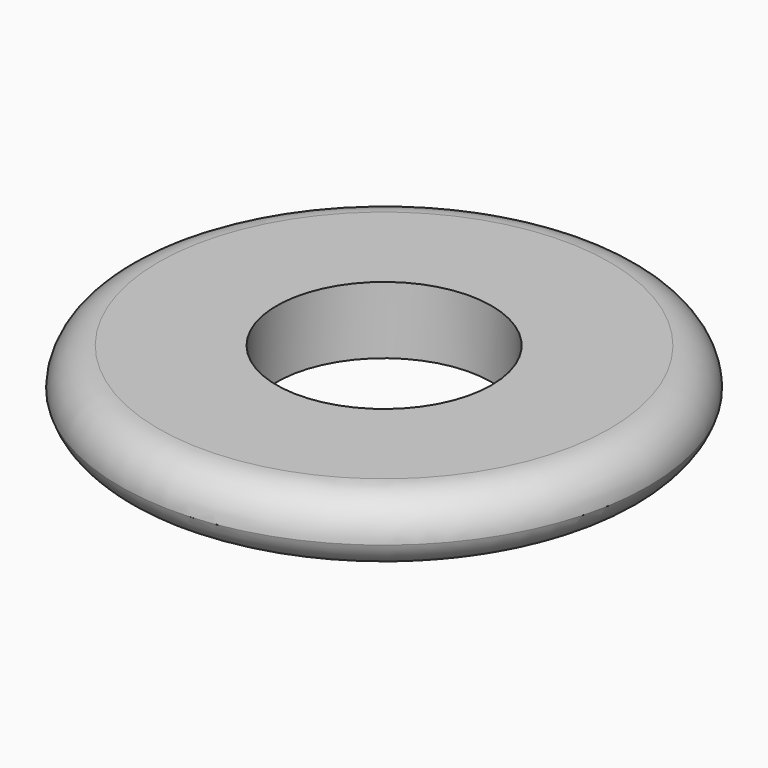
from build123d import *

# Parameters (mm, degrees)
F0_R     = 27.5126478719
F0_R_2   = 11.2
F1_DEPTH = 7
F2_R     = 4


# Not quite as in the source:
# - a fillet or chamfer that OpenCascade refuses, or shapes differently, is made with other operations: its cross-section is extruded or revolved along the edge and cut away or added


with BuildPart() as f1:
    # F0 (on Top) → F1 (new body)
    with BuildSketch(Plane.XY):
        Circle(F0_R)
        Circle(F0_R_2, mode=Mode.SUBTRACT)
    extrude(amount=F1_DEPTH)

    # F2
    f2_edges = [f1.edges().sort_by_distance(p)[0] for p in [
        (-27.512648, 0, 7),
    ]]
    fillet(f2_edges, radius=F2_R)

    # F3: fillet of radius 4 on 1 edges, made by hand

    # F3_s1 → F3_t2 (revolve, cut)
    with BuildSketch(Plane.XZ):
        with BuildLine():
            ThreePointArc((27.5126478719, 3), (26.0891542684, 0.8377223398), (23.6396645256, 0))
            Line((23.6396645256, 0), (27.5126478719, 0))
            Line((27.5126478719, 0), (27.5126478719, 3))
        make_face()
    revolve(axis=Axis((0, 0, 0), (0, 0, 1)), mode=Mode.SUBTRACT)


solid = f1.part
